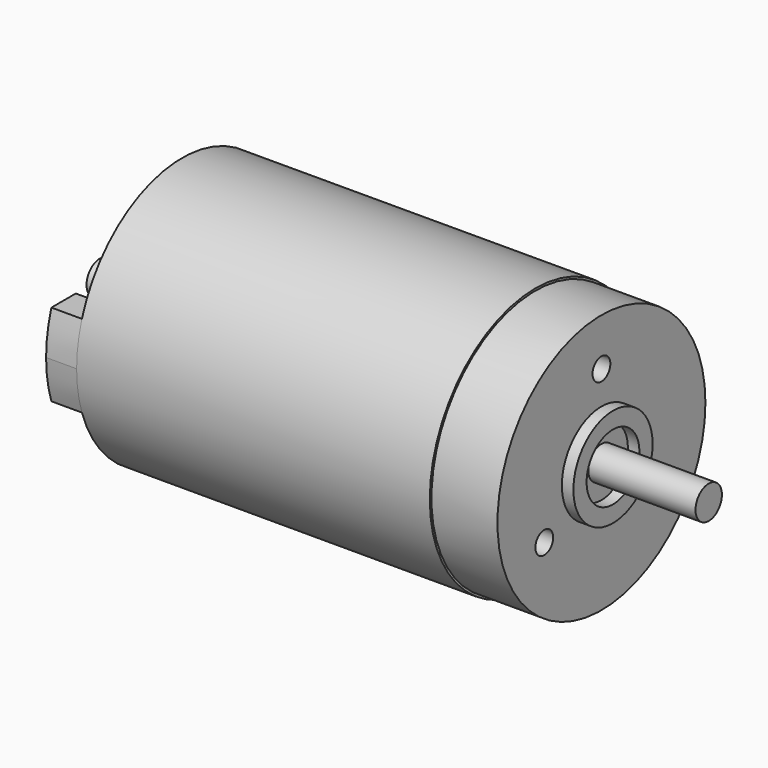
from build123d import *

# Parameters (mm, degrees)
F0_R     = 8
F0_R_2   = 7.875
F0_R_3   = 0.675
F0_R_4   = 3
F0_R_5   = 2
F0_R_6   = 1
F1_DEPTH = 25.4
F2_DEPTH = 6.5
F3_DEPTH = 0.7
F4_DEPTH = 1.35
F5_DEPTH = 4
F6_R     = 1
F7_DEPTH = 5
F6_R_2   = 2.5
F8_DEPTH = 1.85


# Not quite as in the source:
# - after a boolean that leaves OpenCascade's solid faulty, fix() repairs it


with BuildPart() as f1:
    # F0 (on Right) → F1 (new body)
    with BuildSketch(Plane.YZ):
        Circle(F0_R)
        Circle(F0_R_2, mode=Mode.SUBTRACT)
        Circle(F0_R_2)
        with Locations((-4.3301270189, -2.5)):
            Circle(F0_R_3, mode=Mode.SUBTRACT)
        with Locations((4.3301270189, -2.5)):
            Circle(F0_R_3, mode=Mode.SUBTRACT)
        Circle(F0_R_4, mode=Mode.SUBTRACT)
        with Locations((0, 5)):
            Circle(F0_R_3, mode=Mode.SUBTRACT)
        Circle(F0_R_4)
        Circle(F0_R_5, mode=Mode.SUBTRACT)
        Circle(F0_R_5)
        Circle(F0_R_6, mode=Mode.SUBTRACT)
        Circle(F0_R_6)
        with Locations((0, 5)):
            Circle(F0_R_3)
        with Locations((4.3301270189, -2.5)):
            Circle(F0_R_3)
        with Locations((-4.3301270189, -2.5)):
            Circle(F0_R_3)
    extrude(amount=-F1_DEPTH)

    # F0 (on Right) → F2 (join)
    with BuildSketch(Plane.YZ):
        Circle(F0_R_6)
    extrude(amount=F2_DEPTH)

    # F0 (on Right) → F3 (join)
    with BuildSketch(Plane.YZ):
        Circle(F0_R_4)
        Circle(F0_R_5, mode=Mode.SUBTRACT)
    extrude(amount=F3_DEPTH)

    # F0 (on Right) → F4 (cut)
    with BuildSketch(Plane.YZ):
        with Locations((0, 5)):
            Circle(F0_R_3)
        with Locations((4.3301270189, -2.5)):
            Circle(F0_R_3)
        with Locations((-4.3301270189, -2.5)):
            Circle(F0_R_3)
    extrude(amount=-F4_DEPTH, mode=Mode.SUBTRACT)

    # F0 (on Right) → F5 (cut)
    with BuildSketch(Plane.YZ):
        Circle(F0_R)
        Circle(F0_R_2, mode=Mode.SUBTRACT)
    extrude(amount=-F5_DEPTH, mode=Mode.SUBTRACT)

    # F6 (on face) → F7 (join)
    with BuildSketch(Plane(origin=(-25.4, 0, 0), x_dir=(0, -1, 0), z_dir=(-1, 0, 0))):
        Circle(F6_R)
    extrude(amount=F7_DEPTH)

    # F6 (on face) → F8 (join)
    with BuildSketch(Plane(origin=(-25.4, 0, 0), x_dir=(0, -1, 0), z_dir=(-1, 0, 0))):
        Circle(F6_R_2)
        Circle(F6_R, mode=Mode.SUBTRACT)
        with BuildLine():
            ThreePointArc((8, 0), (7.8992004853, 1.2659509046), (7.5993420768, 2.5))
            Line((7.5993420768, 2.5), (5.75, 2.5))
            Line((5.75, 2.5), (5.75, -2.5))
            Line((5.75, -2.5), (7.5993420768, -2.5))
            ThreePointArc((7.5993420768, -2.5), (7.8992004853, -1.2659509046), (8, 0))
        make_face()
        with BuildLine():
            Line((-5.75, 2.5), (-7.5993420768, 2.5))
            ThreePointArc((-7.5993420768, 2.5), (-8, 0), (-7.5993420768, -2.5))
            Line((-7.5993420768, -2.5), (-5.75, -2.5))
            Line((-5.75, -2.5), (-5.75, 2.5))
        make_face()
    extrude(amount=F8_DEPTH)

    add(f1.part.fix(), mode=Mode.REPLACE)


solid = f1.part
